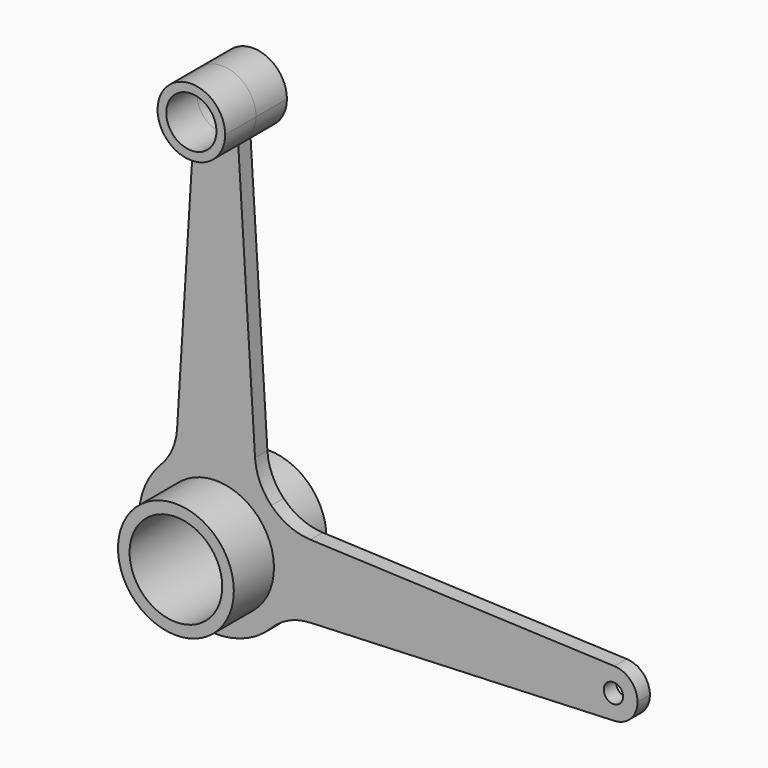
from build123d import *

# Parameters (mm, degrees)
F0_R        = 30
F0_R_2      = 5
F1_DEPTH    = 4
F2_R        = 30
F3_R        = 30
F4_T1_DEPTH = 8
F5_R        = 30
F5_R_2      = 24
F6_DEPTH    = 30
F0_R_3      = 13
F7_DEPTH    = 20


# Not quite as in the source:
# - a fillet or chamfer that OpenCascade refuses, or shapes differently, is made with other operations: its cross-section is extruded or revolved along the edge and cut away or added


with BuildPart() as f1:
    # F0 (on Front) → F1 (new body, symmetric)
    with BuildSketch(Plane.XZ):
        with BuildLine():
            ThreePointArc((34.9249194702, -19.5), (38.7104428986, -10.074800772), (40, 0))
            ThreePointArc((40, 0), (38.7104428986, 10.074800772), (34.9249194702, 19.5))
            ThreePointArc((34.9249194702, 19.5), (28.892590505, 27.6625778609), (21, 34.0440890611))
            ThreePointArc((21, 34.0440890611), (0, 40), (-21, 34.0440890611))
            ThreePointArc((-21, 34.0440890611), (-27.6625778609, -28.892590505), (34.9249194702, -19.5))
        make_face()
        Circle(F0_R, mode=Mode.SUBTRACT)
        with BuildLine():
            ThreePointArc((34.9249194702, 19.5), (38.7104428986, 10.074800772), (40, 0))
            ThreePointArc((40, 0), (38.7104428986, -10.074800772), (34.9249194702, -19.5))
            Line((34.9249194702, -19.5), (206.3684774144, -12.4895628079))
            ThreePointArc((206.3684774144, -12.4895628079), (193.3577711699, 0), (206.3684774144, 12.4895628079))
            Line((206.3684774144, 12.4895628079), (34.9249194702, 19.5))
        make_face()
        with BuildLine():
            ThreePointArc((218.3577711699, 0), (214.8753603171, 8.6563898926), (206.3684774144, 12.4895628079))
            ThreePointArc((206.3684774144, 12.4895628079), (193.3577711699, 0), (206.3684774144, -12.4895628079))
            ThreePointArc((206.3684774144, -12.4895628079), (214.8753603171, -8.6563898926), (218.3577711699, 0))
        make_face()
        with Locations((205.8577711699, 0)):
            Circle(F0_R_2, mode=Mode.SUBTRACT)
        with BuildLine():
            ThreePointArc((-21, 34.0440890611), (0, 40), (21, 34.0440890611))
            Line((21, 34.0440890611), (11.5, 186.8090940417))
            ThreePointArc((11.5, 186.8090940417), (0, 182.5), (-11.5, 186.8090940417))
            Line((-11.5, 186.8090940417), (-21, 34.0440890611))
        make_face()
    extrude(amount=F1_DEPTH, both=True)

    # F2
    f2_edges = [f1.edges().sort_by_distance(p)[0] for p in [
        (-21, 0, 34.044089),
        (34.924919, 0, -19.5),
    ]]
    fillet(f2_edges, radius=F2_R)

    # F3
    f3_edges = [f1.edges().sort_by_distance(p)[0] for p in [
        (34.924919, 0, 19.5),
    ]]
    fillet(f3_edges, radius=F3_R)

    # F4: fillet of radius 30 on 1 edges, made by hand

    # F4_s2 → F4_t1 (join)
    with BuildSketch(Plane.XZ.offset(-4)):
        with BuildLine():
            ThreePointArc((28.649862751, 27.9138919599), (22.7110220839, 36.6919475661), (20.1951004828, 46.9872973509))
            Line((20.1951004828, 46.9872973509), (21, 34.0440890611))
            ThreePointArc((21, 34.0440890611), (25.0134373272, 31.2142267736), (28.649862751, 27.9138919599))
        make_face()
    extrude(amount=F4_T1_DEPTH)

    # F5 (on Front) → F6 (join, symmetric)
    with BuildSketch(Plane.XZ):
        Circle(F5_R)
        Circle(F5_R_2, mode=Mode.SUBTRACT)
    extrude(amount=F6_DEPTH, both=True)

    # F0 (on Front) → F7 (join, symmetric)
    with BuildSketch(Plane.XZ):
        with BuildLine():
            ThreePointArc((-11.5, 186.8090940417), (0, 182.5), (11.5, 186.8090940417))
            ThreePointArc((11.5, 186.8090940417), (15.9295323221, 192.7543116269), (17.5, 200))
            ThreePointArc((17.5, 200), (-7.2456883731, 215.9295323221), (-11.5, 186.8090940417))
        make_face()
        with Locations((0, 200)):
            Circle(F0_R_3, mode=Mode.SUBTRACT)
    extrude(amount=F7_DEPTH, both=True)


solid = f1.part
